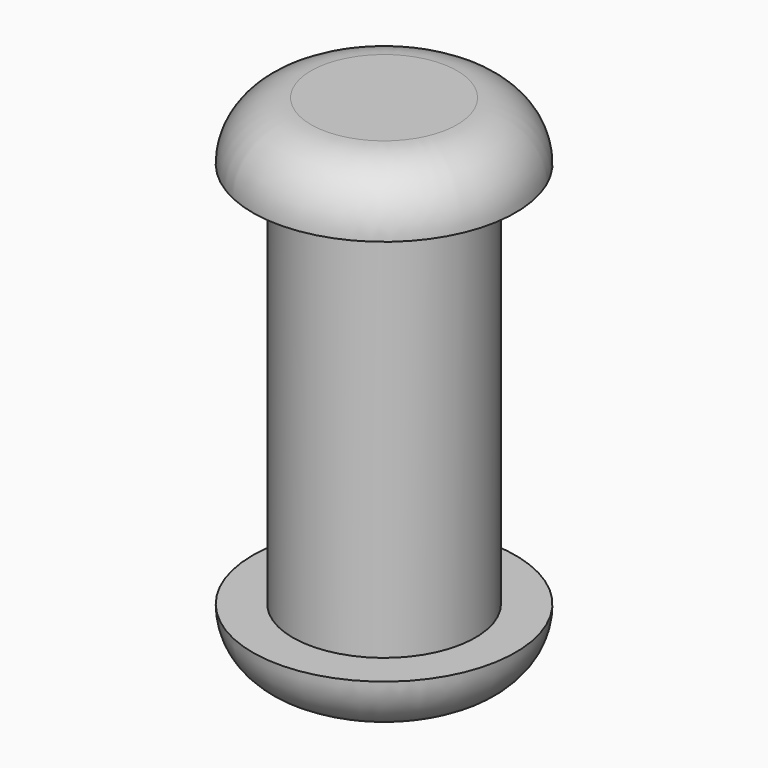
from build123d import *

# Parameters (mm, degrees)
F2_R = 0.79999


# Not quite as in the source:
# - a fillet or chamfer is up to 0.001 mm smaller than in the source, because OpenCascade refuses the exact size


with BuildPart() as f1:
    # F0 (on Front) → F1 (revolve)
    with BuildSketch(Plane.XZ):
        Polygon((-1.8, 2.65), (-1.25, 2.65), (-1.25, -2.65), (-1.8, -2.65), (-1.8, -3.45), (0, -3.45), (0, 0), (0, 3.45), (-1.8, 3.45), align=None)
    revolve(axis=Axis((0, 0, -0.5684057251), (0, 0, -1)))

    # F2 (radius 0.8 in the source; OpenCascade refuses exactly that, so slightly less here)
    f2_edges = [f1.edges().sort_by_distance(p)[0] for p in [
        (1.8, 0, 3.45),
        (1.8, 0, -3.45),
    ]]
    fillet(f2_edges, radius=F2_R)


solid = f1.part
